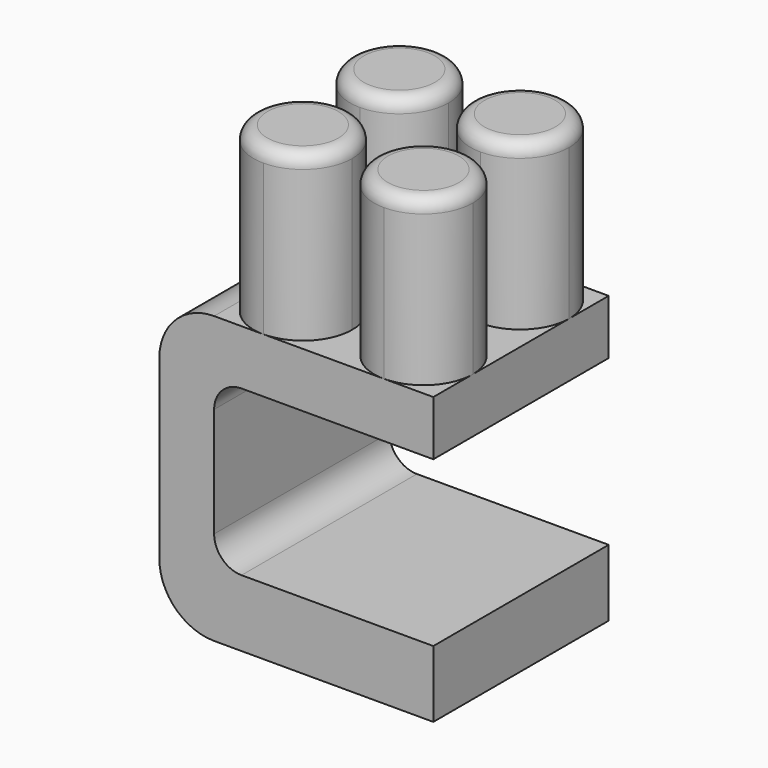
from build123d import *

# Parameters (mm, degrees)
F1_DEPTH = 20
F3_DEPTH = 30


# Not quite as in the source:
# - a fillet or chamfer that OpenCascade refuses, or shapes differently, is made with other operations: its cross-section is extruded or revolved along the edge and cut away or added
# - a feature names something its author has since deleted; it is built from what else it names


with BuildPart() as f1:
    # F0 (on Front) → F1 (new body, symmetric)
    with BuildSketch(Plane.XZ):
        with BuildLine():
            Line((-10, -5), (20, -5))
            Line((20, -5), (20, 5))
            Line((20, 5), (-20, 5))
            ThreePointArc((-20, 5), (-27.0710678119, 2.0710678119), (-30, -5))
            Line((-30, -5), (-30, -37.0084848255))
            Line((-30, -37.0084848255), (-29.9999700785, -37.1900333921))
            ThreePointArc((-29.9999700785, -37.1900333921), (-27.134358967, -44.1955599538), (-20.1815186475, -47.1867371371))
            Line((-20.1815186475, -47.1867371371), (-20, -47.1900331229))
            Line((-20, -47.1900331229), (20, -47.1900331229))
            Line((20, -47.1900331229), (20, -35))
            Line((20, -35), (-15, -35))
            ThreePointArc((-15, -35), (-18.5355339059, -33.5355339059), (-20, -30))
            Line((-20, -30), (-20, -15))
            Line((-20, -15), (-20, -10))
            ThreePointArc((-20, -10), (-18.5355339059, -6.4644660941), (-15, -5))
            Line((-15, -5), (-10, -5))
        make_face()
    extrude(amount=F1_DEPTH, both=True)

    # F2 (on face) → F3 (join)
    with BuildSketch(Plane.XY.offset(5)):
        with BuildLine():
            Line((-11, 11), (-2, 11))
            ThreePointArc((-2, 11), (-4.6360389693, 17.3639610307), (-11, 20))
            Line((-11, 20), (-11, 11))
        make_face()
        with BuildLine():
            Line((-20, 11), (-11, 11))
            Line((-11, 11), (-11, 20))
            ThreePointArc((-11, 20), (-17.3639610307, 17.3639610307), (-20, 11))
        make_face()
        with BuildLine():
            ThreePointArc((-20, 11), (-17.3639610288, 4.6360389675), (-10.9999999948, 2))
            Line((-11, 2), (-11, 11))
            Line((-11, 11), (-20, 11))
        make_face()
        with BuildLine():
            Line((-11, 11), (-11, 2))
            ThreePointArc((-10.9999999948, 2), (-4.6360389675, 4.6360389712), (-2, 11))
            Line((-2, 11), (-11, 11))
        make_face()
        with BuildLine():
            ThreePointArc((11, 20), (4.6360389693, 17.3639610307), (2, 11))
            Line((2, 11), (11, 11))
            Line((11, 11), (11, 20))
        make_face()
        with BuildLine():
            Line((11, 20), (11, 11))
            Line((11, 11), (20, 11))
            ThreePointArc((20, 11), (17.3639610307, 17.3639610307), (11, 20))
        make_face()
        with BuildLine():
            Line((11, 11), (11, 2))
            ThreePointArc((11, 2), (17.3639610307, 4.6360389693), (20, 11))
            Line((20, 11), (11, 11))
        make_face()
        with BuildLine():
            ThreePointArc((2, 11), (4.6360389693, 4.6360389693), (11, 2))
            Line((11, 2), (11, 11))
            Line((11, 11), (2, 11))
        make_face()
        with BuildLine():
            ThreePointArc((11, -2), (4.6360389693, -4.6360389693), (2, -11))
            Line((2, -11), (11, -11))
            Line((11, -11), (11, -2))
        make_face()
        with BuildLine():
            Line((11, -2), (11, -11))
            Line((11, -11), (20, -11))
            ThreePointArc((20, -11), (17.3639610307, -4.6360389693), (11, -2))
        make_face()
        with BuildLine():
            Line((11, -11), (11, -20))
            ThreePointArc((11, -20), (17.3639610307, -17.3639610307), (20, -11))
            Line((20, -11), (11, -11))
        make_face()
        with BuildLine():
            Line((11, -11), (2, -11))
            ThreePointArc((2, -11), (4.6360389693, -17.3639610307), (11, -20))
            Line((11, -20), (11, -11))
        make_face()
        with BuildLine():
            ThreePointArc((-11, -20), (-4.6360389693, -17.3639610307), (-2, -11))
            Line((-2, -11), (-11, -11))
            Line((-11, -11), (-11, -20))
        make_face()
        with BuildLine():
            ThreePointArc((-20, -11), (-17.3639610307, -17.3639610307), (-11, -20))
            Line((-11, -20), (-11, -11))
            Line((-11, -11), (-20, -11))
        make_face()
        with BuildLine():
            Line((-20, -11), (-11, -11))
            Line((-11, -11), (-11, -2))
            ThreePointArc((-11, -2), (-17.3639610307, -4.6360389693), (-20, -11))
        make_face()
        with BuildLine():
            Line((-11, -11), (-2, -11))
            ThreePointArc((-2, -11), (-4.6360389693, -4.6360389693), (-11, -2))
            Line((-11, -2), (-11, -11))
        make_face()
    extrude(amount=F3_DEPTH)

    # F4: fillet of radius 2.5 on 4 edges, made by hand

    # F4_s1 → F4_t2 (revolve, cut)
    with BuildSketch(Plane.YZ.offset(-11)):
        with BuildLine():
            ThreePointArc((2, 32.5), (2.732233047, 34.267766953), (4.5, 35))
            Line((4.5, 35), (2, 35))
            Line((2, 35), (2, 32.5))
        make_face()
    revolve(axis=Axis((-11, 11, 35), (0, 0, 1)), mode=Mode.SUBTRACT)

    # F4_s3 → F4_t4 (revolve, cut)
    with BuildSketch(Plane.XZ.offset(-11)):
        with BuildLine():
            ThreePointArc((2, 32.5), (2.732233047, 34.267766953), (4.5, 35))
            Line((4.5, 35), (2, 35))
            Line((2, 35), (2, 32.5))
        make_face()
    revolve(axis=Axis((11, 11, 35), (0, 0, 1)), mode=Mode.SUBTRACT)

    # F4_s5 → F4_t6 (revolve, cut)
    with BuildSketch(Plane.XZ.offset(11)):
        with BuildLine():
            ThreePointArc((2, 32.5), (2.732233047, 34.267766953), (4.5, 35))
            Line((4.5, 35), (2, 35))
            Line((2, 35), (2, 32.5))
        make_face()
    revolve(axis=Axis((11, -11, 35), (0, 0, 1)), mode=Mode.SUBTRACT)

    # F4_s7 → F4_t8 (revolve, cut)
    with BuildSketch(Plane.XZ.offset(11)):
        with BuildLine():
            ThreePointArc((-2, 32.5), (-2.732233047, 34.267766953), (-4.5, 35))
            Line((-4.5, 35), (-2, 35))
            Line((-2, 35), (-2, 32.5))
        make_face()
    revolve(axis=Axis((-11, -11, 35), (0, 0, 1)), mode=Mode.SUBTRACT)


solid = f1.part
